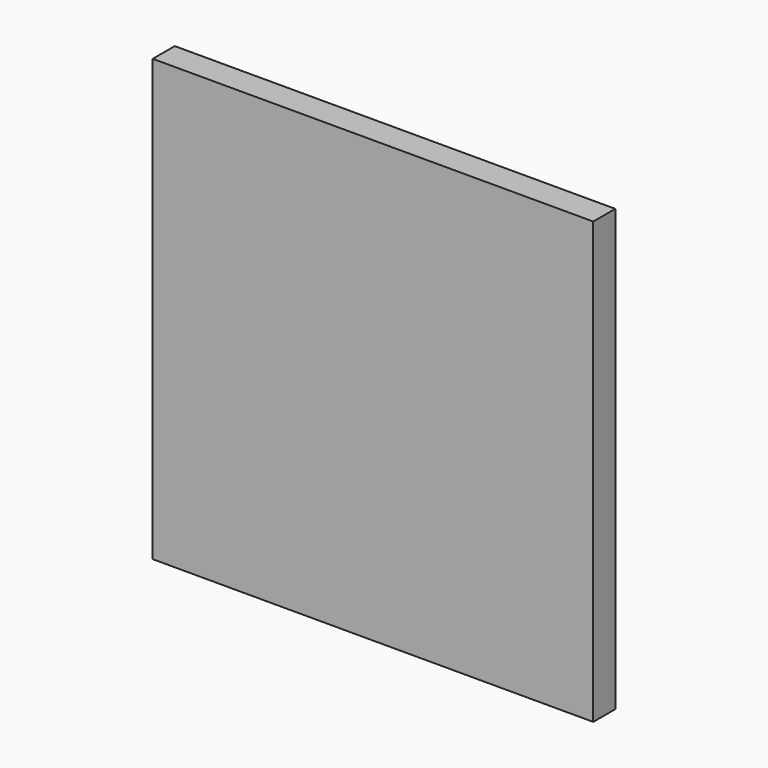
from build123d import *

# Parameters (mm, degrees)
F0_W     = 50.8
F0_H     = 50.8
F1_DEPTH = 3.175


# Not quite as in the source:
# - a length typed as a fraction of an inch, garbled in the dataset ("3 / 203.2 mm" for 3/8 in), is restored


with BuildPart() as f1:
    # F0 (on Front) → F1 (new body)
    with BuildSketch(Plane.XZ):
        Rectangle(F0_W, F0_H)
    extrude(amount=F1_DEPTH)


solid = f1.part
